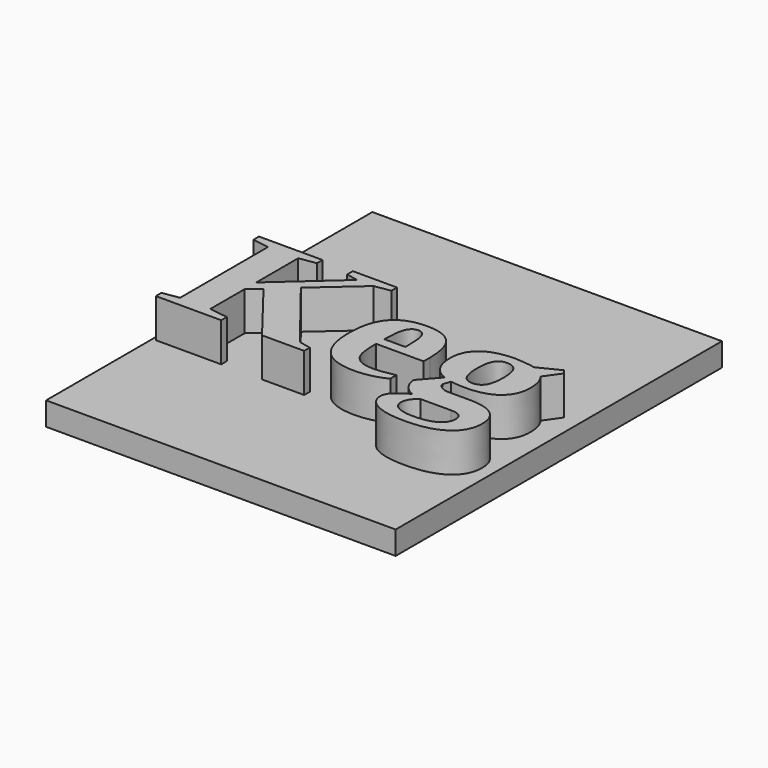
from build123d import *

# Parameters (mm, degrees)
F0_W         = 18
F0_H         = 21
F1_DEPTH     = 1.2
F2_TEXT_SIZE = 10.1435238179
F3_DEPTH     = 2


# Not quite as in the source:
# - Text() gives the source's letters only with a copy of the font that has no kerning and outlines rounded to 1/6400 em; it was checked with that copy


with BuildPart() as f1:
    # F0 (on Top) → F1 (new body)
    with BuildSketch(Plane.XY):
        with Locations((9, 10.5)):
            Rectangle(F0_W, F0_H)
    extrude(amount=F1_DEPTH)

    # F2 (on face) → F3 (join)
    with BuildSketch(Plane.XY.offset(1.2)):
        with Locations((0, 6.8466628511)):
            Text('Keg', F2_TEXT_SIZE, font='Tinos', font_style=FontStyle.BOLD, text_align=(TextAlign.LEFT, TextAlign.BOTTOM))
    extrude(amount=F3_DEPTH)


solid = f1.part
